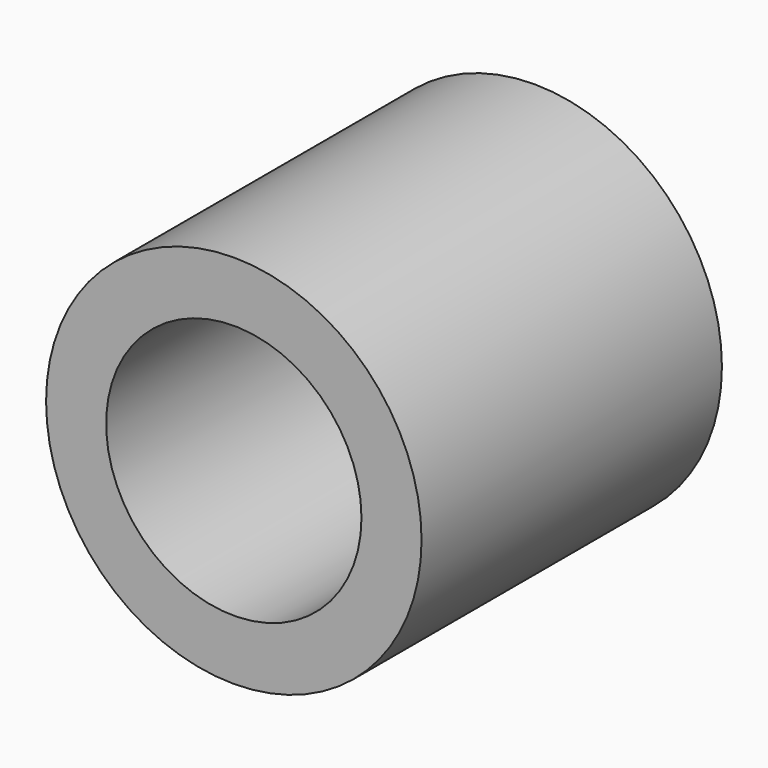
from build123d import *

# Parameters (mm, degrees)
F0_R     = 6.35
F1_DEPTH = 12.7
F2_T     = -2.032
F3_R     = 0.8255
F4_DEPTH = 25.4
F5_R     = 0.8255
F6_DEPTH = 25.4


# Not quite as in the source:
# - a feature names something its author has since deleted; it is built from what else it names


with BuildPart() as f1:
    # F0 (on Front) → F1 (new body)
    with BuildSketch(Plane.XZ):
        with Locations((-39.8430377245, 36.6037674248)):
            Circle(F0_R)
    extrude(amount=F1_DEPTH)

    # F2
    f2_openings = [f1.faces().sort_by_distance(p)[0] for p in [
        (-39.843038, -12.7, 36.603767),
    ]]
    offset(amount=F2_T, openings=f2_openings)

    # F3 (on Front) → F4 (cut)
    with BuildSketch(Plane.XZ):
        with Locations((-40.1724703283, 33.4264033846)):
            Circle(F3_R)
        with Locations((-42.9070014867, 35.9854433805)):
            Circle(F3_R)
        with Locations((-41.3182264228, 39.3769239056)):
            Circle(F3_R)
        with Locations((-37.6017782744, 38.9139341465)):
            Circle(F3_R)
        with Locations((-36.8936620653, 35.2363102138)):
            Circle(F3_R)
    extrude(amount=F4_DEPTH, mode=Mode.SUBTRACT)

    # F5 (on Front) → F6 (cut)
    with BuildSketch(Plane.XZ):
        with Locations((-38.6249683797, 35.9699130058)):
            Circle(F5_R)
        with Locations((-39.3546639971, 38.0343095379)):
            Circle(F5_R)
        with Locations((-41.4190605292, 37.3046139206)):
            Circle(F5_R)
        with Locations((-40.6893649118, 35.2402173885)):
            Circle(F5_R)
    extrude(amount=F6_DEPTH, mode=Mode.SUBTRACT)


solid = f1.part
